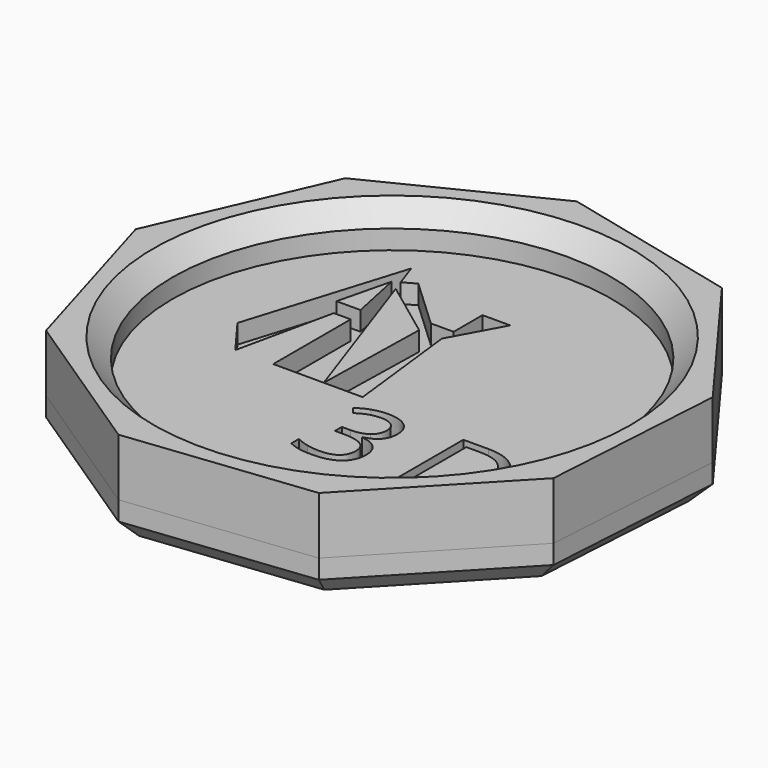
from build123d import *

# Parameters (mm, degrees)
F0_R           = 29.1972530611
F1_DEPTH       = 7.62
F2_DEPTH       = 2.54
F3_SIZE        = 2.54
F0_TEXT_SIZE   = 15.3698635081
F0_TEXT_SIZE_2 = 16.4496738257
F4_DEPTH       = 5.08
F5_SIZE        = 2.54


# Not quite as in the source:
# - Text() gives the source's letters only with a copy of the font that has no kerning and outlines rounded to 1/6400 em; it was checked with that copy


with BuildPart() as f1:
    # F0 (on Top) → F1 (new body)
    with BuildSketch(Plane.XY):
        Polygon((32.9468401064, -14.3677865752), (34.4741789709, 10.1714575329), (19.8706663572, 29.9513636181), (-4.0305518829, 35.7166937941), (-26.0458301024, 24.769785997), (-35.8739749499, 2.2328200464), (-28.9162882234, -21.3489072189), (-8.4283488685, -34.9412435299), (16.0033085927, -32.1841836645), align=None)
        Circle(F0_R, mode=Mode.SUBTRACT)
    extrude(amount=F1_DEPTH)

    # F0 (on Top) → F2 (join)
    with BuildSketch(Plane.XY):
        Circle(F0_R)
        with BuildLine():
            add(Edge.make_bspline(
                [(7.0835487289, -6.9883318099), (8.0319752354, -7.7709764474), (8.0319752354, -9.1357853226)],
                knots=[0, 0, 0, 1, 1, 1], degree=2))
            add(Edge.make_bspline(
                [(8.0319752354, -9.1357853226), (8.0319752354, -10.2615598751), (7.4009760285, -10.9760925819)],
                knots=[0, 0, 0, 1, 1, 1], degree=2))
            add(Edge.make_bspline(
                [(7.4009760285, -10.9760925819), (6.7699768216, -11.6906252887), (5.6133591307, -11.932229873)],
                knots=[0, 0, 0, 1, 1, 1], degree=2))
            Line((5.6133591307, -11.932229873), (5.6133591307, -11.9964864114))
            add(Edge.make_bspline(
                [(5.6133591307, -11.9964864114), (7.0270029751, -12.1712641958), (7.7094074127, -12.894792818)],
                knots=[0, 0, 0, 1, 1, 1], degree=2))
            add(Edge.make_bspline(
                [(7.7094074127, -12.894792818), (8.3918118503, -13.6183214401), (8.3918118503, -14.7903607002)],
                knots=[0, 0, 0, 1, 1, 1], degree=2))
            add(Edge.make_bspline(
                [(8.3918118503, -14.7903607002), (8.3918118503, -16.4687414827), (7.2274833749, -17.3734735432)],
                knots=[0, 0, 0, 1, 1, 1], degree=2))
            add(Edge.make_bspline(
                [(7.2274833749, -17.3734735432), (6.0631548994, -18.2782056036), (3.919556779, -18.2782056036)],
                knots=[0, 0, 0, 1, 1, 1], degree=2))
            add(Edge.make_bspline(
                [(3.919556779, -18.2782056036), (2.9865518417, -18.2782056036), (2.2116179888, -18.1368412191)],
                knots=[0, 0, 0, 1, 1, 1], degree=2))
            add(Edge.make_bspline(
                [(2.2116179888, -18.1368412191), (1.4366841359, -17.9954768347), (0.7067298599, -17.6433510044)],
                knots=[0, 0, 0, 1, 1, 1], degree=2))
            Line((0.7067298599, -17.6433510044), (0.7067298599, -16.3736418059))
            add(Edge.make_bspline(
                [(0.7067298599, -16.3736418059), (1.4700975359, -16.7514702516), (2.3337054117, -16.9480952591)],
                knots=[0, 0, 0, 1, 1, 1], degree=2))
            add(Edge.make_bspline(
                [(2.3337054117, -16.9480952591), (3.1973132876, -17.1447202665), (3.9683917482, -17.1447202665)],
                knots=[0, 0, 0, 1, 1, 1], degree=2))
            add(Edge.make_bspline(
                [(3.9683917482, -17.1447202665), (7.0115814059, -17.1447202665), (7.0115814059, -14.7595175618)],
                knots=[0, 0, 0, 1, 1, 1], degree=2))
            add(Edge.make_bspline(
                [(7.0115814059, -14.7595175618), (7.0115814059, -12.6210599645), (3.6548198409, -12.6210599645)],
                knots=[0, 0, 0, 1, 1, 1], degree=2))
            Line((3.6548198409, -12.6210599645), (2.49820215, -12.6210599645))
            Line((2.49820215, -12.6210599645), (2.49820215, -11.4747233197))
            Line((2.49820215, -11.4747233197), (3.6702414101, -11.4747233197))
            add(Edge.make_bspline(
                [(3.6702414101, -11.4747233197), (5.0427610699, -11.4747233197), (5.8459677997, -10.8681415974)],
                knots=[0, 0, 0, 1, 1, 1], degree=2))
            add(Edge.make_bspline(
                [(5.8459677997, -10.8681415974), (6.6491745294, -10.2615598751), (6.6491745294, -9.1846202918)],
                knots=[0, 0, 0, 1, 1, 1], degree=2))
            add(Edge.make_bspline(
                [(6.6491745294, -9.1846202918), (6.6491745294, -8.326152939), (6.0592995071, -7.8352329858)],
                knots=[0, 0, 0, 1, 1, 1], degree=2))
            add(Edge.make_bspline(
                [(6.0592995071, -7.8352329858), (5.4694244847, -7.3443130326), (4.4567414399, -7.3443130326)],
                knots=[0, 0, 0, 1, 1, 1], degree=2))
            add(Edge.make_bspline(
                [(4.4567414399, -7.3443130326), (3.6856629793, -7.3443130326), (3.0032585417, -7.5537893477)],
                knots=[0, 0, 0, 1, 1, 1], degree=2))
            add(Edge.make_bspline(
                [(3.0032585417, -7.5537893477), (2.3208541041, -7.7632656628), (1.4443949205, -8.326152939)],
                knots=[0, 0, 0, 1, 1, 1], degree=2))
            Line((1.4443949205, -8.326152939), (0.7709863983, -7.4265614017))
            add(Edge.make_bspline(
                [(0.7709863983, -7.4265614017), (1.4932298897, -6.8559633409), (2.4365158731, -6.5308252567)],
                knots=[0, 0, 0, 1, 1, 1], degree=2))
            add(Edge.make_bspline(
                [(2.4365158731, -6.5308252567), (3.3798018566, -6.2056871724), (4.4258983014, -6.2056871724)],
                knots=[0, 0, 0, 1, 1, 1], degree=2))
            add(Edge.make_bspline(
                [(4.4258983014, -6.2056871724), (6.1351222224, -6.2056871724), (7.0835487289, -6.9883318099)],
                knots=[0, 0, 0, 1, 1, 1], degree=2))
        make_face(mode=Mode.SUBTRACT)
        with BuildLine():
            add(Edge.make_bspline(
                [(21.4838249545, -7.2677888518), (22.9019350172, -8.6858989145), (22.9019350172, -11.2315325581)],
                knots=[0, 0, 0, 1, 1, 1], degree=2))
            add(Edge.make_bspline(
                [(22.9019350172, -11.2315325581), (22.9019350172, -13.9476756249), (21.4273887369, -15.384998017)],
                knots=[0, 0, 0, 1, 1, 1], degree=2))
            add(Edge.make_bspline(
                [(21.4273887369, -15.384998017), (19.9528424566, -16.8223204091), (17.183865484, -16.8223204091)],
                knots=[0, 0, 0, 1, 1, 1], degree=2))
            Line((17.183865484, -16.8223204091), (14.1435143588, -16.8223204091))
            Line((14.1435143588, -16.8223204091), (14.1435143588, -5.8496787891))
            Line((14.1435143588, -5.8496787891), (17.5056720012, -5.8496787891))
            add(Edge.make_bspline(
                [(17.5056720012, -5.8496787891), (20.0657148917, -5.8496787891), (21.4838249545, -7.2677888518)],
                knots=[0, 0, 0, 1, 1, 1], degree=2))
        make_face(mode=Mode.SUBTRACT)
        Polygon((-16.9251915067, -4.8957169056), (-20.5620117486, 0), (-14.1276400536, 20.8417661488), (-13.0433699584, 17.7244897167), (-11.4301005378, 18.6333339661), (-4.8284097575, 12.4645419419), (-1.7981252167, 12.4645419419), (-1.7981252167, 17.2582045197), (1.8815047806, 17.2582045197), (-1.7981252167, 10.5165019631), (0, -4.8957169056), (-5.1754717715, -4.8957169056), (-11.889597401, -4.8957169056), (-11.889597401, 7.9730246216), (-14.1276400536, 7.9730246216), align=None, mode=Mode.SUBTRACT)
    extrude(amount=F2_DEPTH)

    # F0 (on Top) → F2, piece 2 (join)
    with BuildSketch(Plane.XY):
        Polygon((-4.8284097575, 10.5165019631), (-12.5346167738, 16.2618243539), (-5.1754717715, -4.8957169056), align=None)
    extrude(amount=F2_DEPTH)

    # F3
    f3_edges = [f1.edges().sort_by_distance(p)[0] for p in [
        (-29.197253, 0, 7.62),
    ]]
    chamfer(f3_edges, length=F3_SIZE)


with BuildPart() as f2:
    # F0 (on Top) → F2, piece 3 (new body)
    with BuildSketch(Plane.XY):
        Polygon((-12.402520515, 10.2418372408), (-13.871062547, 17.2582045197), (-15.5843617395, 10.2418372408), align=None)
    extrude(amount=F2_DEPTH)


with BuildPart() as f2b:
    # F0 (on Top) → F2, piece 4 (new body)
    with BuildSketch(Plane.XY):
        with BuildLine():
            add(Edge.make_bspline(
                [(20.4031314266, -14.5972925122), (21.5522688779, -13.4745720138), (21.5522688779, -11.2771618404)],
                knots=[0, 0, 0, 1, 1, 1], degree=2))
            add(Edge.make_bspline(
                [(21.5522688779, -11.2771618404), (21.5522688779, -9.1301840316), (20.4751776618, -8.0422858801)],
                knots=[0, 0, 0, 1, 1, 1], degree=2))
            add(Edge.make_bspline(
                [(20.4751776618, -8.0422858801), (19.3980864456, -6.9543877287), (17.2727225074, -6.9543877287)],
                knots=[0, 0, 0, 1, 1, 1], degree=2))
            Line((17.2727225074, -6.9543877287), (15.4187327217, -6.9543877287))
            Line((15.4187327217, -6.9543877287), (15.4187327217, -15.7200130107))
            Line((15.4187327217, -15.7200130107), (16.9725298607, -15.7200130107))
            add(Edge.make_bspline(
                [(16.9725298607, -15.7200130107), (19.2539939752, -15.7200130107), (20.4031314266, -14.5972925122)],
                knots=[0, 0, 0, 1, 1, 1], degree=2))
        make_face()
    extrude(amount=F2_DEPTH)


with BuildPart() as f4:
    # F0 (on Top) → F4 (new body)
    with BuildSketch(Plane.XY):
        Polygon((32.9468401064, -14.3677865752), (34.4741789709, 10.1714575329), (19.8706663572, 29.9513636181), (-4.0305518829, 35.7166937941), (-26.0458301024, 24.769785997), (-35.8739749499, 2.2328200464), (-28.9162882234, -21.3489072189), (-8.4283488685, -34.9412435299), (16.0033085927, -32.1841836645), align=None)
        Circle(F0_R, mode=Mode.SUBTRACT)
        Circle(F0_R)
        with BuildLine():
            add(Edge.make_bspline(
                [(7.0835487289, -6.9883318099), (8.0319752354, -7.7709764474), (8.0319752354, -9.1357853226)],
                knots=[0, 0, 0, 1, 1, 1], degree=2))
            add(Edge.make_bspline(
                [(8.0319752354, -9.1357853226), (8.0319752354, -10.2615598751), (7.4009760285, -10.9760925819)],
                knots=[0, 0, 0, 1, 1, 1], degree=2))
            add(Edge.make_bspline(
                [(7.4009760285, -10.9760925819), (6.7699768216, -11.6906252887), (5.6133591307, -11.932229873)],
                knots=[0, 0, 0, 1, 1, 1], degree=2))
            Line((5.6133591307, -11.932229873), (5.6133591307, -11.9964864114))
            add(Edge.make_bspline(
                [(5.6133591307, -11.9964864114), (7.0270029751, -12.1712641958), (7.7094074127, -12.894792818)],
                knots=[0, 0, 0, 1, 1, 1], degree=2))
            add(Edge.make_bspline(
                [(7.7094074127, -12.894792818), (8.3918118503, -13.6183214401), (8.3918118503, -14.7903607002)],
                knots=[0, 0, 0, 1, 1, 1], degree=2))
            add(Edge.make_bspline(
                [(8.3918118503, -14.7903607002), (8.3918118503, -16.4687414827), (7.2274833749, -17.3734735432)],
                knots=[0, 0, 0, 1, 1, 1], degree=2))
            add(Edge.make_bspline(
                [(7.2274833749, -17.3734735432), (6.0631548994, -18.2782056036), (3.919556779, -18.2782056036)],
                knots=[0, 0, 0, 1, 1, 1], degree=2))
            add(Edge.make_bspline(
                [(3.919556779, -18.2782056036), (2.9865518417, -18.2782056036), (2.2116179888, -18.1368412191)],
                knots=[0, 0, 0, 1, 1, 1], degree=2))
            add(Edge.make_bspline(
                [(2.2116179888, -18.1368412191), (1.4366841359, -17.9954768347), (0.7067298599, -17.6433510044)],
                knots=[0, 0, 0, 1, 1, 1], degree=2))
            Line((0.7067298599, -17.6433510044), (0.7067298599, -16.3736418059))
            add(Edge.make_bspline(
                [(0.7067298599, -16.3736418059), (1.4700975359, -16.7514702516), (2.3337054117, -16.9480952591)],
                knots=[0, 0, 0, 1, 1, 1], degree=2))
            add(Edge.make_bspline(
                [(2.3337054117, -16.9480952591), (3.1973132876, -17.1447202665), (3.9683917482, -17.1447202665)],
                knots=[0, 0, 0, 1, 1, 1], degree=2))
            add(Edge.make_bspline(
                [(3.9683917482, -17.1447202665), (7.0115814059, -17.1447202665), (7.0115814059, -14.7595175618)],
                knots=[0, 0, 0, 1, 1, 1], degree=2))
            add(Edge.make_bspline(
                [(7.0115814059, -14.7595175618), (7.0115814059, -12.6210599645), (3.6548198409, -12.6210599645)],
                knots=[0, 0, 0, 1, 1, 1], degree=2))
            Line((3.6548198409, -12.6210599645), (2.49820215, -12.6210599645))
            Line((2.49820215, -12.6210599645), (2.49820215, -11.4747233197))
            Line((2.49820215, -11.4747233197), (3.6702414101, -11.4747233197))
            add(Edge.make_bspline(
                [(3.6702414101, -11.4747233197), (5.0427610699, -11.4747233197), (5.8459677997, -10.8681415974)],
                knots=[0, 0, 0, 1, 1, 1], degree=2))
            add(Edge.make_bspline(
                [(5.8459677997, -10.8681415974), (6.6491745294, -10.2615598751), (6.6491745294, -9.1846202918)],
                knots=[0, 0, 0, 1, 1, 1], degree=2))
            add(Edge.make_bspline(
                [(6.6491745294, -9.1846202918), (6.6491745294, -8.326152939), (6.0592995071, -7.8352329858)],
                knots=[0, 0, 0, 1, 1, 1], degree=2))
            add(Edge.make_bspline(
                [(6.0592995071, -7.8352329858), (5.4694244847, -7.3443130326), (4.4567414399, -7.3443130326)],
                knots=[0, 0, 0, 1, 1, 1], degree=2))
            add(Edge.make_bspline(
                [(4.4567414399, -7.3443130326), (3.6856629793, -7.3443130326), (3.0032585417, -7.5537893477)],
                knots=[0, 0, 0, 1, 1, 1], degree=2))
            add(Edge.make_bspline(
                [(3.0032585417, -7.5537893477), (2.3208541041, -7.7632656628), (1.4443949205, -8.326152939)],
                knots=[0, 0, 0, 1, 1, 1], degree=2))
            Line((1.4443949205, -8.326152939), (0.7709863983, -7.4265614017))
            add(Edge.make_bspline(
                [(0.7709863983, -7.4265614017), (1.4932298897, -6.8559633409), (2.4365158731, -6.5308252567)],
                knots=[0, 0, 0, 1, 1, 1], degree=2))
            add(Edge.make_bspline(
                [(2.4365158731, -6.5308252567), (3.3798018566, -6.2056871724), (4.4258983014, -6.2056871724)],
                knots=[0, 0, 0, 1, 1, 1], degree=2))
            add(Edge.make_bspline(
                [(4.4258983014, -6.2056871724), (6.1351222224, -6.2056871724), (7.0835487289, -6.9883318099)],
                knots=[0, 0, 0, 1, 1, 1], degree=2))
        make_face(mode=Mode.SUBTRACT)
        with BuildLine():
            add(Edge.make_bspline(
                [(21.4838249545, -7.2677888518), (22.9019350172, -8.6858989145), (22.9019350172, -11.2315325581)],
                knots=[0, 0, 0, 1, 1, 1], degree=2))
            add(Edge.make_bspline(
                [(22.9019350172, -11.2315325581), (22.9019350172, -13.9476756249), (21.4273887369, -15.384998017)],
                knots=[0, 0, 0, 1, 1, 1], degree=2))
            add(Edge.make_bspline(
                [(21.4273887369, -15.384998017), (19.9528424566, -16.8223204091), (17.183865484, -16.8223204091)],
                knots=[0, 0, 0, 1, 1, 1], degree=2))
            Line((17.183865484, -16.8223204091), (14.1435143588, -16.8223204091))
            Line((14.1435143588, -16.8223204091), (14.1435143588, -5.8496787891))
            Line((14.1435143588, -5.8496787891), (17.5056720012, -5.8496787891))
            add(Edge.make_bspline(
                [(17.5056720012, -5.8496787891), (20.0657148917, -5.8496787891), (21.4838249545, -7.2677888518)],
                knots=[0, 0, 0, 1, 1, 1], degree=2))
        make_face(mode=Mode.SUBTRACT)
        Polygon((-16.9251915067, -4.8957169056), (-20.5620117486, 0), (-14.1276400536, 20.8417661488), (-13.0433699584, 17.7244897167), (-11.4301005378, 18.6333339661), (-4.8284097575, 12.4645419419), (-1.7981252167, 12.4645419419), (-1.7981252167, 17.2582045197), (1.8815047806, 17.2582045197), (-1.7981252167, 10.5165019631), (0, -4.8957169056), (-5.1754717715, -4.8957169056), (-11.889597401, -4.8957169056), (-11.889597401, 7.9730246216), (-14.1276400536, 7.9730246216), align=None, mode=Mode.SUBTRACT)
        Polygon((-14.1276400536, 20.8417661488), (-20.5620117486, 0), (-16.9251915067, -4.8957169056), (-14.1276400536, 7.9730246216), (-11.889597401, 7.9730246216), (-11.889597401, -4.8957169056), (-5.1754717715, -4.8957169056), (-12.5346167738, 16.2618243539), (-13.871062547, 17.2582045197), (-13.0433699584, 17.7244897167), align=None)
        Polygon((-15.5843617395, 10.2418372408), (-13.871062547, 17.2582045197), (-12.402520515, 10.2418372408), align=None, mode=Mode.SUBTRACT)
        Polygon((-11.4301005378, 18.6333339661), (-13.0433699584, 17.7244897167), (-12.5346167738, 16.2618243539), (-4.8284097575, 10.5165019631), (-5.1754717715, -4.8957169056), (0, -4.8957169056), (-1.7981252167, 10.5165019631), (1.8815047806, 17.2582045197), (-1.7981252167, 17.2582045197), (-1.7981252167, 12.4645419419), (-4.8284097575, 12.4645419419), align=None)
        with Locations((12.6353465021, -16.8223204091)):
            Text('D', F0_TEXT_SIZE, font='Open Sans', text_align=(TextAlign.LEFT, TextAlign.BOTTOM))
        Polygon((-4.8284097575, 10.5165019631), (-12.5346167738, 16.2618243539), (-5.1754717715, -4.8957169056), align=None)
        with BuildLine():
            add(Edge.make_bspline(
                [(20.4031314266, -14.5972925122), (21.5522688779, -13.4745720138), (21.5522688779, -11.2771618404)],
                knots=[0, 0, 0, 1, 1, 1], degree=2))
            add(Edge.make_bspline(
                [(21.5522688779, -11.2771618404), (21.5522688779, -9.1301840316), (20.4751776618, -8.0422858801)],
                knots=[0, 0, 0, 1, 1, 1], degree=2))
            add(Edge.make_bspline(
                [(20.4751776618, -8.0422858801), (19.3980864456, -6.9543877287), (17.2727225074, -6.9543877287)],
                knots=[0, 0, 0, 1, 1, 1], degree=2))
            Line((17.2727225074, -6.9543877287), (15.4187327217, -6.9543877287))
            Line((15.4187327217, -6.9543877287), (15.4187327217, -15.7200130107))
            Line((15.4187327217, -15.7200130107), (16.9725298607, -15.7200130107))
            add(Edge.make_bspline(
                [(16.9725298607, -15.7200130107), (19.2539939752, -15.7200130107), (20.4031314266, -14.5972925122)],
                knots=[0, 0, 0, 1, 1, 1], degree=2))
        make_face()
        with Locations((-0.0489270315, -18.1162791268)):
            Text('3', F0_TEXT_SIZE_2, font='Open Sans', text_align=(TextAlign.LEFT, TextAlign.BOTTOM))
        Polygon((-12.402520515, 10.2418372408), (-13.871062547, 17.2582045197), (-15.5843617395, 10.2418372408), align=None)
    extrude(amount=-F4_DEPTH)

    # F5
    f5_edges = [f4.edges().sort_by_distance(p)[0] for p in [
        (33.71051, -2.098165, -5.08),
        (24.475074, -23.275985, -5.08),
        (3.78748, -33.562714, -5.08),
        (-18.672319, -28.145075, -5.08),
        (-32.395132, -9.558044, -5.08),
        (-30.959903, 13.501303, -5.08),
        (-15.038191, 30.24324, -5.08),
        (7.920057, 32.834029, -5.08),
        (27.172423, 20.061411, -5.08),
    ]]
    chamfer(f5_edges, length=F5_SIZE)


solid = Compound([f1.part, f2.part, f2b.part, f4.part])
